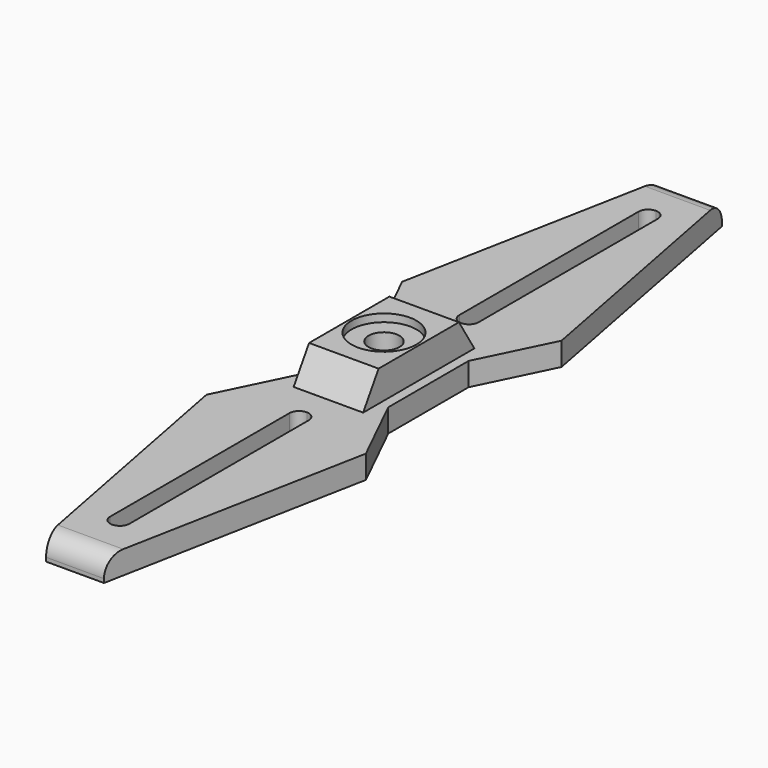
from build123d import *

# Parameters (mm, degrees)
F1_DEPTH  = 6
F2_W      = 18
F2_H      = 36
F3_DEPTH  = 8
F4_SIZE2  = 7.99999
F4_SIZE   = 4.99999
F6_DEPTH  = 1
F7_R      = 8.4004464167
F8_DEPTH  = 2
F9_R      = 4
F10_DEPTH = 25
F11_R     = 5


# Not quite as in the source:
# - a fillet or chamfer is up to 0.001 mm smaller than in the source, because OpenCascade refuses the exact size


with BuildPart() as f1:
    # F0 (on Top) → F1 (new body)
    with BuildSketch(Plane.XY):
        Polygon((7.5, 100), (-7.5, 100), (-20.6415709108, 31.671449542), (-11.5, 13), (-11.5, -13), (-20.6415709108, -31.671449542), (-7.5, -100), (7.5, -100), (20.6415709108, -31.671449542), (11.5, -13), (11.5, 13), (20.6415709108, 31.671449542), align=None)
        with BuildLine():
            ThreePointArc((0, -88), (-1.767766953, -87.267766953), (-2.5, -85.5))
            Line((-2.5, -85.5), (-2.5, -27.5))
            ThreePointArc((-2.5, -27.5), (-1.767766953, -25.732233047), (0, -25))
            ThreePointArc((0, -25), (1.767766953, -25.732233047), (2.5, -27.5))
            Line((2.5, -27.5), (2.5, -85.5))
            ThreePointArc((2.5, -85.5), (1.767766953, -87.267766953), (0, -88))
        make_face(mode=Mode.SUBTRACT)
        Polygon((-6.5, 3.7527767497), (0, 7.5055534995), (6.5, 3.7527767497), (6.5, -3.7527767497), (0, -7.5055534995), (-6.5, -3.7527767497), align=None, mode=Mode.SUBTRACT)
        with BuildLine():
            ThreePointArc((0, 25), (-1.767766953, 25.732233047), (-2.5, 27.5))
            Line((-2.5, 27.5), (-2.5, 85.5))
            ThreePointArc((-2.5, 85.5), (-1.767766953, 87.267766953), (0, 88))
            ThreePointArc((0, 88), (1.767766953, 87.267766953), (2.5, 85.5))
            Line((2.5, 85.5), (2.5, 27.5))
            ThreePointArc((2.5, 27.5), (1.767766953, 25.732233047), (0, 25))
        make_face(mode=Mode.SUBTRACT)
    extrude(amount=F1_DEPTH)

    # F2 (on face) → F3 (join)
    with BuildSketch(Plane.XY.offset(6)):
        Rectangle(F2_W, F2_H)
    extrude(amount=F3_DEPTH)

    # F4 (size 5 and 8 in the source; OpenCascade refuses exactly that, so slightly less here)
    f4_edges = [f1.edges().sort_by_distance(p)[0] for p in [
        (0, -18, 14),
        (0, 18, 14),
    ]]
    f4_side = f1.faces().sort_by_distance((0, 0, 14))[0]
    chamfer(f4_edges, length=F4_SIZE, length2=F4_SIZE2, reference=f4_side)

    # F5 (on face) → F6 (cut)
    with BuildSketch(Plane(origin=(0, 0, 6), x_dir=(1, 0, 0), z_dir=(0, 0, -1))):
        Polygon((6.5, 3.7527767497), (0, 7.5055534995), (-6.5, 3.7527767497), (-6.5, -3.7527767497), (0, -7.5055534995), (6.5, -3.7527767497), align=None)
    extrude(amount=-F6_DEPTH, mode=Mode.SUBTRACT)

    # F7 (on face) → F8 (cut)
    with BuildSketch(Plane.XY.offset(14)):
        Circle(F7_R)
    extrude(amount=-F8_DEPTH, mode=Mode.SUBTRACT)

    # F9 (on face) → F10 (cut)
    with BuildSketch(Plane.XY.offset(12)):
        Circle(F9_R)
    extrude(amount=-F10_DEPTH, mode=Mode.SUBTRACT)

    # F11
    f11_edges = [f1.edges().sort_by_distance(p)[0] for p in [
        (0, -100, 6),
        (0, 100, 6),
    ]]
    fillet(f11_edges, radius=F11_R)


solid = f1.part
